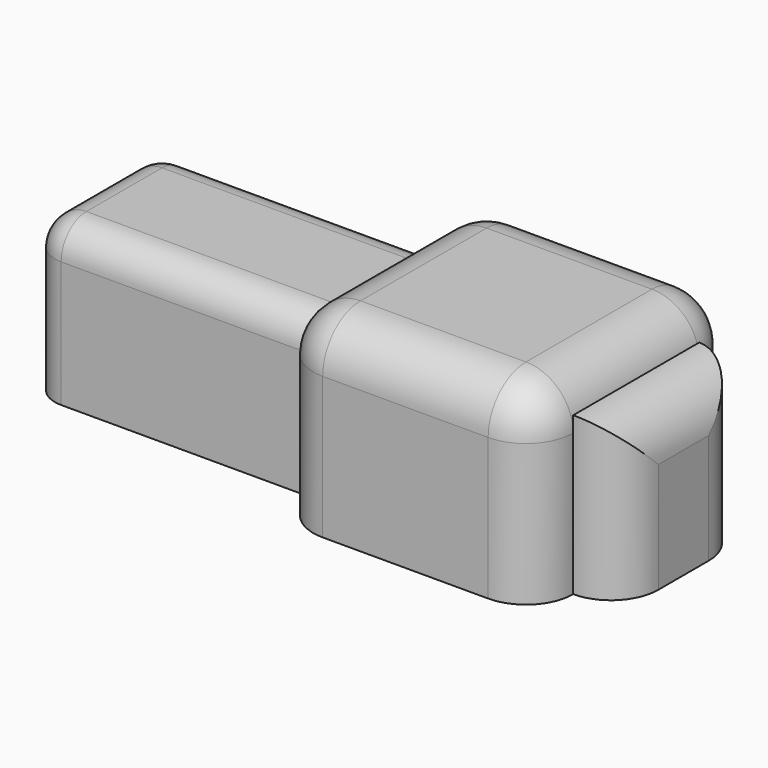
from build123d import *

# Parameters (mm, degrees)
F0_W     = 18.0000008929
F0_H     = 10
F1_DEPTH = 10
F0_W_2   = 3
F2_DEPTH = 12
F3_R     = 2
F4_R     = 3
F5_R     = 2.99999
F7_DEPTH = 10


# Not quite as in the source:
# - a fillet or chamfer is up to 0.001 mm smaller than in the source, because OpenCascade refuses the exact size


with BuildPart() as f1:
    # F0 (on Top) → F1 (new body)
    with BuildSketch(Plane.XY):
        with Locations((-18.9999995536, 5)):
            Rectangle(F0_W, F0_H)
    extrude(amount=F1_DEPTH)

    # F3
    f3_edges = [f1.edges().sort_by_distance(p)[0] for p in [
        (-19, 0, 10),
        (-28, 0, 5),
        (-28, 5, 10),
        (-28, 10, 5),
        (-19, 10, 10),
    ]]
    fillet(f3_edges, radius=F3_R)

    # F6 (on face) → F7 (cut)
    with BuildSketch(Plane(origin=(-28, 0, 0), x_dir=(0, -1, 0), z_dir=(-1, 0, 0))):
        with BuildLine():
            ThreePointArc((-8, 4.2267539538), (-5, 1.2267539538), (-2, 4.2267539538))
            ThreePointArc((-2, 4.2267539538), (-5, 7.2267539538), (-8, 4.2267539538))
        make_face()
    extrude(amount=-F7_DEPTH, mode=Mode.SUBTRACT)


with BuildPart() as f1b:
    # F0 (on Top) → F1, piece 2 (new body)
    with BuildSketch(Plane.XY):
        with Locations((7.9999984374, 5)):
            Rectangle(F0_W_2, F0_H)
    extrude(amount=F1_DEPTH)

    # F5 (radius 3 in the source; OpenCascade refuses exactly that, so slightly less here)
    f5_edges = [f1b.edges().sort_by_distance(p)[0] for p in [
        (9.499998, 5, 10),
        (9.499998, 0, 5),
        (9.499998, 10, 5),
    ]]
    fillet(f5_edges, radius=F5_R)


with BuildPart() as f2:
    # F0 (on Top) → F2 (new body)
    with BuildSketch(Plane.XY):
        Polygon((-9.9999991071, 10), (-9.9999991071, 0), (-9.9999991071, -3.0000002232), (6.4999984374, -3.0000002232), (6.4999984374, 0), (6.4999984374, 10), (6.4999984374, 13.0000013393), (-9.9999991071, 13.0000013393), align=None)
    extrude(amount=F2_DEPTH)

    # F4
    f4_edges = [f2.edges().sort_by_distance(p)[0] for p in [
        (-9.999999, 5.000001, 12),
        (-1.75, -3, 12),
        (6.499998, 5.000001, 12),
        (-1.75, 13.000001, 12),
        (6.499998, -3, 6),
        (-9.999999, -3, 6),
        (-9.999999, 13.000001, 6),
        (6.499998, 13.000001, 6),
    ]]
    fillet(f4_edges, radius=F4_R)


solid = Compound([f1.part, f1b.part, f2.part])
